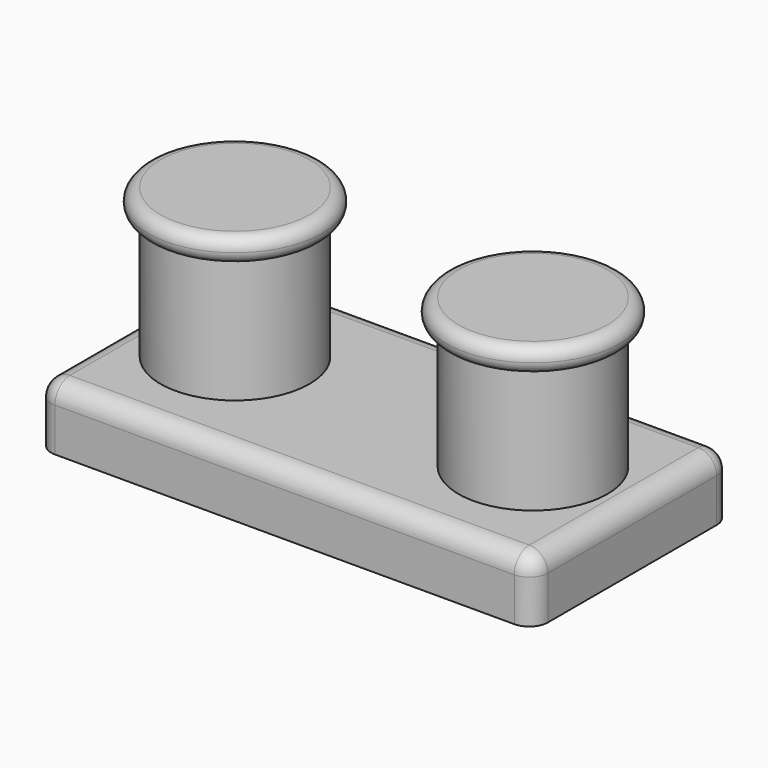
from build123d import *

# Parameters (mm, degrees)
F0_W     = 40
F0_H     = 20
F1_DEPTH = 5
F2_R     = 6
F3_DEPTH = 10
F4_R     = 7
F5_DEPTH = 2
F6_R     = 7
F7_DEPTH = 2
F8_R     = 1.5
F9_R     = 0.99999


# Not quite as in the source:
# - a fillet or chamfer is up to 0.001 mm smaller than in the source, because OpenCascade refuses the exact size


with BuildPart() as f1:
    # F0 (on Top) → F1 (new body)
    with BuildSketch(Plane.XY):
        Rectangle(F0_W, F0_H)
    extrude(amount=F1_DEPTH)

    # F2 (on face) → F3 (join)
    with BuildSketch(Plane.XY.offset(5)):
        with Locations((-12, 0)):
            Circle(F2_R)
        with Locations((12, 0)):
            Circle(F2_R)
    extrude(amount=F3_DEPTH)

    # F4 (on face) → F5 (join)
    with BuildSketch(Plane.XY.offset(15)):
        with Locations((-12, 0)):
            Circle(F4_R)
    extrude(amount=F5_DEPTH)

    # F6 (on face) → F7 (join)
    with BuildSketch(Plane.XY.offset(15)):
        with Locations((12, 0)):
            Circle(F6_R)
    extrude(amount=F7_DEPTH)

    # F8
    f8_edges = [f1.edges().sort_by_distance(p)[0] for p in [
        (0, -10, 5),
        (-20, 0, 5),
        (0, 10, 5),
        (20, 0, 5),
        (20, -10, 2.5),
        (20, 10, 2.5),
        (-20, 10, 2.5),
        (-20, -10, 2.5),
    ]]
    fillet(f8_edges, radius=F8_R)

    # F9 (radius 1 in the source; OpenCascade refuses exactly that, so slightly less here)
    f9_edges = [f1.edges().sort_by_distance(p)[0] for p in [
        (-19, 0, 15),
        (5, 0, 15),
        (-19, 0, 17),
        (5, 0, 17),
    ]]
    fillet(f9_edges, radius=F9_R)


solid = f1.part
